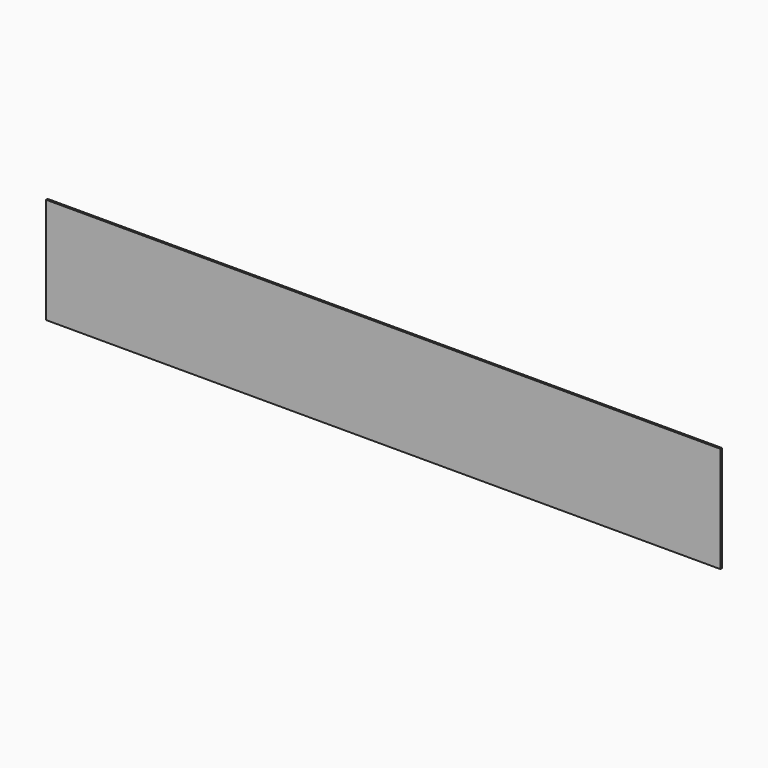
from build123d import *

# Parameters (mm, degrees)
F0_W     = 1930.4
F0_H     = 303.2125
F1_DEPTH = 5.55625


# Not quite as in the source:
# - a length typed as a fraction of an inch, garbled in the dataset ("3 / 203.2 mm" for 3/8 in), is restored


with BuildPart() as f1:
    # F0 (on Front) → F1 (new body)
    with BuildSketch(Plane.XZ):
        with Locations((851.4691745162, 126.579282251)):
            Rectangle(F0_W, F0_H)
    extrude(amount=F1_DEPTH)


solid = f1.part
